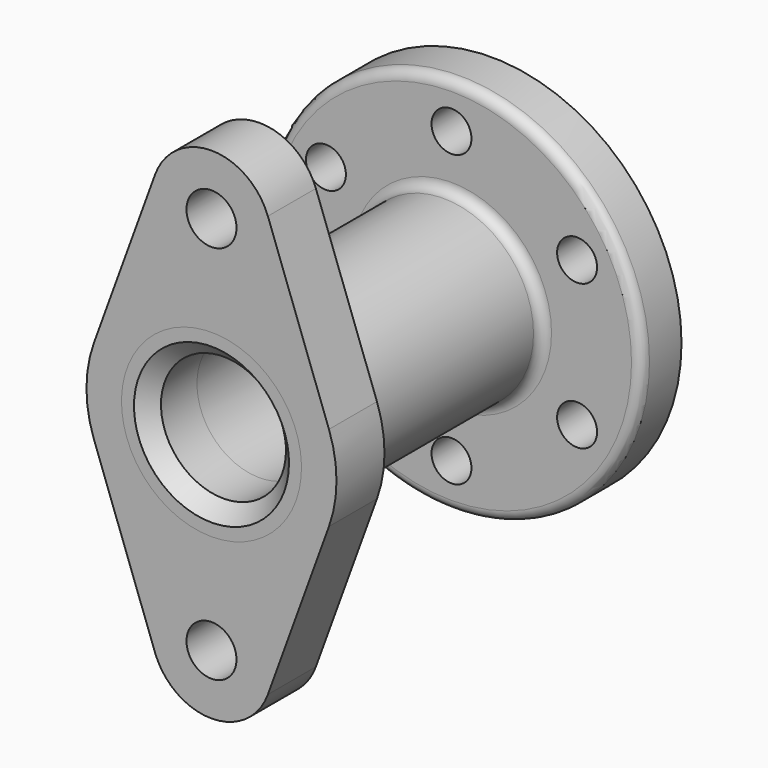
from build123d import *

# Parameters (mm, degrees)
F0_R      = 965.2
F1_DEPTH  = 254
F2_D      = 202.946
F3_R      = 457.2
F3_R_2    = 317.5
F4_DEPTH  = 1219.2
F5_R      = 50.8
F3_R_3    = 254
F6_DEPTH  = 254.001
F7_DEPTH  = 584.2
F10_DEPTH = 304.8
F11_DEPTH = 304.8
F12_SIZE2 = 76.2
F12_SIZE  = 76.2


# Not quite as in the source:
# - a feature names something its author has since deleted; it is built from what else it names


with BuildPart() as f1:
    # F0 (on Front) → F1 (new body)
    with BuildSketch(Plane.XZ):
        Circle(F0_R)
        with BuildLine():
            ThreePointArc((682.5252094596, 277.017866666), (722.9549188186, 141.1231566967), (736.6, 0))
            ThreePointArc((736.6, 0), (722.9549188186, -141.1231566967), (682.5252094596, -277.017866666))
            ThreePointArc((682.5252094596, -277.017866666), (724.0973360995, -314.4943643214), (739.5143124276, -368.3))
            ThreePointArc((739.5143124276, -368.3), (685.6481824631, -457.9885592004), (581.1671145647, -452.5752367823))
            ThreePointArc((581.1671145647, -452.5752367823), (368.3, -637.9143124276), (101.3580948948, -729.5931034483))
            ThreePointArc((101.3580948949, -729.5931034483), (101.5395057141, -733.0944644715), (101.6, -736.6))
            ThreePointArc((101.6, -736.6), (-3.5055355285, -838.1395057141), (-101.3580948949, -729.5931034483))
            ThreePointArc((-101.3580948948, -729.5931034483), (-368.3, -637.9143124276), (-581.1671145647, -452.5752367823))
            ThreePointArc((-581.1671145647, -452.5752367823), (-725.9024934521, -419.1), (-682.5252094596, -277.017866666))
            ThreePointArc((-682.5252094596, -277.017866666), (-736.6, 0), (-682.5252094596, 277.017866666))
            ThreePointArc((-682.5252094596, 277.017866666), (-725.9024934521, 419.1), (-581.1671145647, 452.5752367823))
            ThreePointArc((-581.1671145647, 452.5752367823), (-368.3, 637.9143124276), (-101.3580948948, 729.5931034483))
            ThreePointArc((-101.3580948949, 729.5931034483), (-3.5055355285, 838.1395057141), (101.6, 736.6))
            ThreePointArc((101.6, 736.6), (101.5395057141, 733.0944644715), (101.3580948949, 729.5931034483))
            ThreePointArc((101.3580948948, 729.5931034483), (368.3, 637.9143124276), (581.1671145647, 452.5752367823))
            ThreePointArc((581.1671145647, 452.5752367823), (685.6481824631, 457.9885592004), (739.5143124276, 368.3))
            ThreePointArc((739.5143124276, 368.3), (724.0973360995, 314.4943643214), (682.5252094596, 277.017866666))
        make_face(mode=Mode.SUBTRACT)
        with BuildLine():
            ThreePointArc((682.5252094596, -277.017866666), (722.9549188186, -141.1231566967), (736.6, 0))
            ThreePointArc((736.6, 0), (722.9549188186, 141.1231566967), (682.5252094596, 277.017866666))
            ThreePointArc((682.5252094596, 277.017866666), (549.9261314031, 317.5), (581.1671145647, 452.5752367823))
            ThreePointArc((581.1671145647, 452.5752367823), (368.3, 637.9143124276), (101.3580948948, 729.5931034483))
            ThreePointArc((101.3580948949, 729.5931034483), (0, 635), (-101.3580948949, 729.5931034483))
            ThreePointArc((-101.3580948948, 729.5931034483), (-368.3, 637.9143124276), (-581.1671145647, 452.5752367823))
            ThreePointArc((-581.1671145647, 452.5752367823), (-548.2257532273, 416.0338700355), (-536.3143124276, 368.3))
            ThreePointArc((-536.3143124276, 368.3), (-584.108676749, 282.1169763282), (-682.5252094596, 277.017866666))
            ThreePointArc((-682.5252094596, 277.017866666), (-736.6, 0), (-682.5252094596, -277.017866666))
            ThreePointArc((-682.5252094596, -277.017866666), (-584.108676749, -282.1169763282), (-536.3143124276, -368.3))
            ThreePointArc((-536.3143124276, -368.3), (-548.2257532273, -416.0338700355), (-581.1671145647, -452.5752367823))
            ThreePointArc((-581.1671145647, -452.5752367823), (-368.3, -637.9143124276), (-101.3580948948, -729.5931034483))
            ThreePointArc((-101.3580948949, -729.5931034483), (0, -635), (101.3580948949, -729.5931034483))
            ThreePointArc((101.3580948948, -729.5931034483), (368.3, -637.9143124276), (581.1671145647, -452.5752367823))
            ThreePointArc((581.1671145647, -452.5752367823), (549.9261314031, -317.5), (682.5252094596, -277.017866666))
        make_face()
        with BuildLine():
            ThreePointArc((-682.5252094596, 277.017866666), (-637.9143124276, 368.3), (-581.1671145647, 452.5752367823))
            ThreePointArc((-581.1671145647, 452.5752367823), (-725.9024934521, 419.1), (-682.5252094596, 277.017866666))
        make_face()
        with BuildLine():
            ThreePointArc((-101.3580948948, 729.5931034483), (0, 736.6), (101.3580948948, 729.5931034483))
            ThreePointArc((101.3580948949, 729.5931034483), (101.5395057141, 733.0944644715), (101.6, 736.6))
            ThreePointArc((101.6, 736.6), (-3.5055355285, 838.1395057141), (-101.3580948949, 729.5931034483))
        make_face()
        with BuildLine():
            ThreePointArc((-682.5252094596, -277.017866666), (-725.9024934521, -419.1), (-581.1671145647, -452.5752367823))
            ThreePointArc((-581.1671145647, -452.5752367823), (-637.9143124276, -368.3), (-682.5252094596, -277.017866666))
        make_face()
        with BuildLine():
            ThreePointArc((101.6, -736.6), (101.5395057141, -733.0944644715), (101.3580948949, -729.5931034483))
            ThreePointArc((101.3580948948, -729.5931034483), (0, -736.6), (-101.3580948948, -729.5931034483))
            ThreePointArc((-101.3580948949, -729.5931034483), (-3.5055355285, -838.1395057141), (101.6, -736.6))
        make_face()
        with BuildLine():
            ThreePointArc((739.5143124276, -368.3), (724.0973360995, -314.4943643214), (682.5252094596, -277.017866666))
            ThreePointArc((682.5252094596, -277.017866666), (637.9143124276, -368.3), (581.1671145647, -452.5752367823))
            ThreePointArc((581.1671145647, -452.5752367823), (685.6481824631, -457.9885592004), (739.5143124276, -368.3))
        make_face()
        with BuildLine():
            ThreePointArc((581.1671145647, 452.5752367823), (637.9143124276, 368.3), (682.5252094596, 277.017866666))
            ThreePointArc((682.5252094596, 277.017866666), (724.0973360995, 314.4943643214), (739.5143124276, 368.3))
            ThreePointArc((739.5143124276, 368.3), (685.6481824631, 457.9885592004), (581.1671145647, 452.5752367823))
        make_face()
        with BuildLine():
            ThreePointArc((-536.3143124276, 368.3), (-548.2257532273, 416.0338700355), (-581.1671145647, 452.5752367823))
            ThreePointArc((-581.1671145647, 452.5752367823), (-637.9143124276, 368.3), (-682.5252094596, 277.017866666))
            ThreePointArc((-682.5252094596, 277.017866666), (-584.108676749, 282.1169763282), (-536.3143124276, 368.3))
        make_face()
        with BuildLine():
            ThreePointArc((-101.3580948949, 729.5931034483), (0, 635), (101.3580948949, 729.5931034483))
            ThreePointArc((101.3580948948, 729.5931034483), (0, 736.6), (-101.3580948948, 729.5931034483))
        make_face()
        with BuildLine():
            ThreePointArc((-682.5252094596, -277.017866666), (-637.9143124276, -368.3), (-581.1671145647, -452.5752367823))
            ThreePointArc((-581.1671145647, -452.5752367823), (-548.2257532273, -416.0338700355), (-536.3143124276, -368.3))
            ThreePointArc((-536.3143124276, -368.3), (-584.108676749, -282.1169763282), (-682.5252094596, -277.017866666))
        make_face()
        with BuildLine():
            ThreePointArc((-101.3580948948, -729.5931034483), (0, -736.6), (101.3580948948, -729.5931034483))
            ThreePointArc((101.3580948949, -729.5931034483), (0, -635), (-101.3580948949, -729.5931034483))
        make_face()
        with BuildLine():
            ThreePointArc((581.1671145647, -452.5752367823), (637.9143124276, -368.3), (682.5252094596, -277.017866666))
            ThreePointArc((682.5252094596, -277.017866666), (549.9261314031, -317.5), (581.1671145647, -452.5752367823))
        make_face()
        with BuildLine():
            ThreePointArc((581.1671145647, 452.5752367823), (549.9261314031, 317.5), (682.5252094596, 277.017866666))
            ThreePointArc((682.5252094596, 277.017866666), (637.9143124276, 368.3), (581.1671145647, 452.5752367823))
        make_face()
    extrude(amount=F1_DEPTH)

    # F2 (through all)
    with Locations(Plane(origin=(0, 0, 0), x_dir=(1, 0, 0), z_dir=(0, 1, 0))):
        with Locations((0, -736.6), (-637.9143124276, -368.3), (-637.9143124276, 368.3), (0, 736.6), (637.9143124276, 368.3), (637.9143124276, -368.3)):
            Hole(F2_D / 2)

    # F3 (on face) → F4 (join)
    with BuildSketch(Plane.XZ.offset(254)):
        Circle(F3_R)
        Circle(F3_R_2, mode=Mode.SUBTRACT)
    extrude(amount=F4_DEPTH)

    # F5
    f5_edges = [f1.edges().sort_by_distance(p)[0] for p in [
        (-965.2, -254, 0),
        (-457.2, -254, 0),
    ]]
    fillet(f5_edges, radius=F5_R)

    # F3 (on face) → F6 (cut, through all)
    with BuildSketch(Plane.XZ.offset(254)):
        Circle(F3_R_3)
    extrude(amount=-F6_DEPTH, mode=Mode.SUBTRACT)

    # F3 (on face) → F7 (join)
    with BuildSketch(Plane.XZ.offset(254)):
        Circle(F3_R_2)
        Circle(F3_R_3, mode=Mode.SUBTRACT)
    extrude(amount=F7_DEPTH)

    # F9 (on face) → F10 (join)
    with BuildSketch(Plane.XZ.offset(1473.2)):
        with BuildLine():
            ThreePointArc((0, 660.4), (215.5261469057, 749.6738530943), (304.8, 965.2))
            ThreePointArc((304.8, 965.2), (300.1670055935, 1018.1415597902), (286.40886645, 1069.4736842105))
            ThreePointArc((286.40886645, 1069.4736842105), (0, 1270), (-286.40886645, 1069.4736842105))
            ThreePointArc((-286.40886645, 1069.4736842105), (-249.6854610779, 790.3852107906), (0, 660.4))
        make_face()
        with BuildLine():
            ThreePointArc((127, 965.2), (89.8025612107, 875.3974387893), (0, 838.2))
            ThreePointArc((0, 838.2), (-89.8025612107, 1055.0025612107), (127, 965.2))
        make_face(mode=Mode.SUBTRACT)
        with BuildLine():
            ThreePointArc((286.40886645, 1069.4736842105), (300.1670055935, 1018.1415597902), (304.8, 965.2))
            ThreePointArc((304.8, 965.2), (215.5261469057, 749.6738530943), (0, 660.4))
            Line((0, 660.4), (0, 635))
            ThreePointArc((0, 635), (364.1974814541, 520.1780411576), (596.6851417238, 217.2368330788))
            Line((596.6851417238, 217.2368330788), (286.40886645, 1069.4736842105))
        make_face()
        with BuildLine():
            Line((0, 635), (0, 660.4))
            ThreePointArc((0, 660.4), (-249.6854610779, 790.3852107906), (-286.40886645, 1069.4736842105))
            Line((-286.40886645, 1069.4736842105), (-596.6851384375, 217.2368421053))
            ThreePointArc((-596.6851384375, 217.2368421053), (-364.1974775195, 520.1780439123), (0, 635))
        make_face()
        with BuildLine():
            ThreePointArc((635, 0), (625.3479291541, 110.2949114996), (596.6851417238, 217.2368330788))
            ThreePointArc((596.6851417238, 217.2368330788), (364.1974814541, 520.1780411576), (0, 635))
            Line((0, 635), (0, 457.2))
            Line((0, 457.2), (0, 330.2))
            ThreePointArc((0, 330.2), (233.4866591478, 233.4866591478), (330.2, 0))
            ThreePointArc((330.2, 0), (233.4866591478, -233.4866591478), (0, -330.2))
            Line((0, -330.2), (0, -635))
            ThreePointArc((0, -635), (364.1974775195, -520.1780439123), (596.6851384375, -217.2368421053))
            ThreePointArc((596.6851384375, -217.2368421053), (625.3479283198, -110.2949162297), (635, 0))
        make_face()
        with BuildLine():
            Line((0, 457.2), (0, 635))
            ThreePointArc((0, 635), (-364.1974775195, 520.1780439123), (-596.6851384375, 217.2368421053))
            ThreePointArc((-596.6851384375, 217.2368421053), (-635, 4.0958e-06), (-596.6851412398, -217.236834408))
            ThreePointArc((-596.6851412398, -217.236834408), (-364.1974808747, -520.1780415632), (0, -635))
            Line((0, -635), (0, -330.2))
            ThreePointArc((0, -330.2), (-233.4866591478, -233.4866591478), (-330.2, 0))
            Line((-330.2, 0), (-457.2, 0))
            ThreePointArc((-457.2, 0), (-323.2892203585, 323.2892203585), (0, 457.2))
        make_face()
        with BuildLine():
            Line((0, 330.2), (0, 457.2))
            ThreePointArc((0, 457.2), (-323.2892203585, 323.2892203585), (-457.2, 0))
            Line((-457.2, 0), (-330.2, 0))
            ThreePointArc((-330.2, 0), (-233.4866591478, 233.4866591478), (0, 330.2))
        make_face()
        with BuildLine():
            ThreePointArc((0, -635), (-364.1974808747, -520.1780415632), (-596.6851412398, -217.236834408))
            Line((-596.6851412398, -217.236834408), (-286.40886645, -1069.4736842105))
            ThreePointArc((-286.40886645, -1069.4736842105), (-249.6854610779, -790.3852107906), (0, -660.4))
            Line((0, -660.4), (0, -635))
        make_face()
        with BuildLine():
            Line((286.4088669044, -1069.4736829624), (596.6851384375, -217.2368421053))
            ThreePointArc((596.6851384375, -217.2368421053), (364.1974775195, -520.1780439123), (0, -635))
            Line((0, -635), (0, -660.4))
            ThreePointArc((0, -660.4), (215.5261469057, -749.6738530943), (304.8, -965.2))
            ThreePointArc((304.8, -965.2), (300.1670057089, -1018.1415591362), (286.4088669044, -1069.4736829624))
        make_face()
        with BuildLine():
            ThreePointArc((0, -660.4), (-249.6854610779, -790.3852107906), (-286.40886645, -1069.4736842105))
            ThreePointArc((-286.40886645, -1069.4736842105), (6.642e-07, -1270), (286.4088669044, -1069.4736829624))
            ThreePointArc((286.4088669044, -1069.4736829624), (300.1670057089, -1018.1415591362), (304.8, -965.2))
            ThreePointArc((304.8, -965.2), (215.5261469057, -749.6738530943), (0, -660.4))
        make_face()
        with BuildLine():
            ThreePointArc((127, -965.2), (-89.8025612107, -1055.0025612107), (0, -838.2))
            ThreePointArc((0, -838.2), (89.8025612107, -875.3974387893), (127, -965.2))
        make_face(mode=Mode.SUBTRACT)
    extrude(amount=F10_DEPTH)

    # F8 (on face) → F11 (join)
    with BuildSketch(Plane.XZ.offset(1473.2)):
        with BuildLine():
            Line((0, -457.2), (0, -317.5))
            ThreePointArc((0, -317.5), (-224.5064030267, -224.5064030267), (-317.5, 0))
            Line((-317.5, 0), (-457.2, 0))
            ThreePointArc((-457.2, 0), (-323.2892203585, -323.2892203585), (0, -457.2))
        make_face()
        with BuildLine():
            ThreePointArc((-317.5, 0), (-224.5064030267, 224.5064030267), (0, 317.5))
            Line((0, 317.5), (0, 457.2))
            ThreePointArc((0, 457.2), (-323.2892203585, 323.2892203585), (-457.2, 0))
            Line((-457.2, 0), (-317.5, 0))
        make_face()
        with BuildLine():
            Line((0, 457.2), (0, 317.5))
            ThreePointArc((0, 317.5), (224.5064030267, 224.5064030267), (317.5, 0))
            Line((317.5, 0), (457.2, 0))
            ThreePointArc((457.2, 0), (323.2892203585, 323.2892203585), (0, 457.2))
        make_face()
        with BuildLine():
            ThreePointArc((317.5, 0), (224.5064030267, -224.5064030267), (0, -317.5))
            Line((0, -317.5), (0, -457.2))
            ThreePointArc((0, -457.2), (323.2892203585, -323.2892203585), (457.2, 0))
            Line((457.2, 0), (317.5, 0))
        make_face()
    extrude(amount=F11_DEPTH)

    # F12
    f12_edges = [f1.edges().sort_by_distance(p)[0] for p in [
        (-317.5, -1778, 0),
    ]]
    chamfer(f12_edges, length=F12_SIZE, length2=F12_SIZE2)


solid = f1.part
